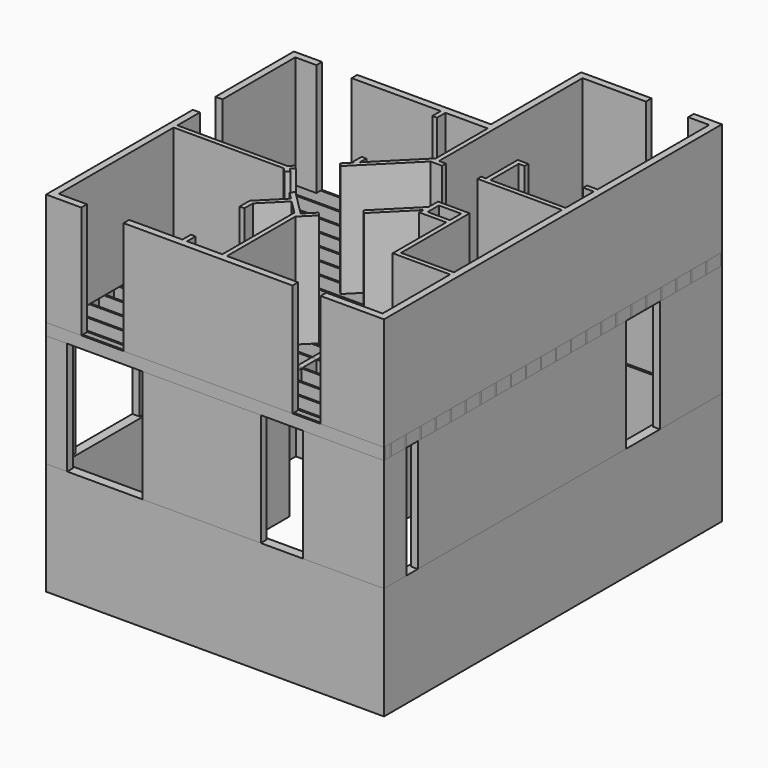
from build123d import *

# Parameters (mm, degrees)
F3_DEPTH  = 2438.4
F5_DEPTH  = 2438.4
F4_W      = 101.6
F4_H      = 1651.1016
F4_W_2    = 482.6
F4_H_2    = 304.8
F6_W      = 114.3
F6_H      = 254
F7_DEPTH  = 9144
F6_W_2    = 38.1
F8_W      = 38.1
F8_H      = 254
F9_DEPTH  = 7315.2
F11_DEPTH = 2438.4
F10_W     = 482.6
F10_H     = 304.8
F13_DEPTH = 5130.801


with BuildPart() as f3:
    # F2 (on Top) → F3 (new body)
    with BuildSketch(Plane.XY):
        Polygon((-4267.2, 0), (0, 0), (3048, 0), (3048, 9144), (0, 9144), (0, 6705.6), (-4267.2, 6705.6), align=None)
        Polygon((-4064, 6502.4), (203.2, 6502.4), (203.2, 8940.8), (2844.8, 8940.8), (2844.8, 203.2), (0, 203.2), (-4064, 203.2), align=None, mode=Mode.SUBTRACT)
    extrude(amount=-F3_DEPTH)


with BuildPart() as f5:
    # F4 (on face) → F5 (new body)
    with BuildSketch(Plane.XY):
        Polygon((-4267.2, 152.4), (-4267.2, 0), (-3810, 0), (-3810, 152.4), (-4114.8, 152.4), (-4114.8, 609.6), (-4267.2, 609.6), align=None)
    extrude(amount=F5_DEPTH)


with BuildPart() as f5b:
    # F4 (on face) → F5, piece 2 (new body)
    with BuildSketch(Plane.XY):
        Polygon((-4267.2, 6705.6), (-4267.2, 2336.8), (-4114.8, 2336.8), (-4114.8, 5232.4), (-3149.6, 5232.4), (-3149.6, 5334), (-4114.8, 5334), (-4114.8, 6553.2), (-2286, 6553.2), (-2286, 5334), (-2387.6, 5334), (-2387.6, 5232.4), (-2184.4, 5232.4), (-2184.4, 5334), (-2184.4, 6553.2), (-1879.6, 6553.2), (-1879.6, 6705.6), (-4114.8, 6705.6), align=None)
    extrude(amount=F5_DEPTH)


with BuildPart() as f5c:
    # F4 (on face) → F5, piece 3 (new body)
    with BuildSketch(Plane.XY):
        Polygon((0, 6705.6), (-1066.8, 6705.6), (-1066.8, 6553.2), (0, 6553.2), (152.4, 6553.2), (152.4, 8991.6), (2895.6, 8991.6), (2895.6, 7467.6), (3048, 7467.6), (3048, 8991.6), (3048, 9144), (152.4, 9144), (0, 9144), align=None)
    extrude(amount=F5_DEPTH)


with BuildPart() as f5d:
    # F4 (on face) → F5, piece 4 (new body)
    with BuildSketch(Plane.XY):
        Polygon((3048, 914.4), (3048, 6553.2), (2895.6, 6553.2), (2895.6, 5181.6), (1752.6, 5181.6), (1752.6, 5080.1016), (2895.6, 5080.1016), (2895.6, 914.4), align=None)
    extrude(amount=F5_DEPTH)


with BuildPart() as f5e:
    # F4 (on face) → F5, piece 5 (new body)
    with BuildSketch(Plane.XY):
        Polygon((-2184.4, 152.4), (-2184.4, 0), (381, 0), (381, 152.4), (152.4, 152.4), (152.4, 1066.8), (50.8, 1066.8), (50.8, 152.4), align=None)
    extrude(amount=F5_DEPTH)


with BuildPart() as f5f:
    # F4 (on face) → F5, piece 6 (new body)
    with BuildSketch(Plane.XY):
        Polygon((2895.6, 152.4), (1295.4, 152.4), (1295.4, 0), (3048, 0), (3048, 152.4), (3048, 609.6), (2895.6, 609.6), align=None)
    extrude(amount=F5_DEPTH)


with BuildPart() as f5g:
    # F4 (on face) → F5, piece 7 (new body)
    with BuildSketch(Plane.XY):
        with Locations((101.6, 3111.5508)):
            Rectangle(F4_W, F4_H)
    extrude(amount=F5_DEPTH)


with BuildPart() as f5h:
    # F4 (on face) → F5, piece 8 (new body)
    with BuildSketch(Plane.XY):
        Polygon((1752.6, 3937.1016), (1066.8, 3937.1016), (1066.8, 3276.8032), (1168.4, 3276.8032), (1168.4, 3429.2032), (1651, 3429.2032), (1651, 1473.2), (1168.4, 1473.2), (1168.4, 1655.9784), (1066.8, 1655.9784), (1066.8, 1371.6), (1752.6, 1371.6), align=None)
        with Locations((1409.7, 3683.1016)):
            Rectangle(F4_W_2, F4_H_2, mode=Mode.SUBTRACT)
    extrude(amount=F5_DEPTH)


with BuildPart() as f7:
    # F6 (on Front) → F7 (new body)
    with BuildSketch(Plane.XZ):
        with Locations((95.25, 2565.4)):
            Rectangle(F6_W, F6_H)
    extrude(amount=-F7_DEPTH)


with BuildPart() as f7b:
    # F6 (on Front) → F7, piece 2 (new body)
    with BuildSketch(Plane.XZ):
        with Locations((3028.95, 2565.4)):
            Rectangle(F6_W_2, F6_H)
    extrude(amount=-F7_DEPTH)


with BuildPart() as f7c:
    # F6 (on Front) → F7, piece 3 (new body)
    with BuildSketch(Plane.XZ):
        with Locations((-4248.15, 2565.4)):
            Rectangle(F6_W_2, F6_H)
    extrude(amount=-F7_DEPTH)

    # F8 (on face) → F9, piece 7 (join)
    with BuildSketch(Plane(origin=(-4267.2, 0, 0), x_dir=(0, -1, 0), z_dir=(-1, 0, 0))):
        with Locations((-6686.55, 2565.4)):
            Rectangle(F8_W, F8_H)
        with Locations((-6280.15, 2565.4)):
            Rectangle(F8_W, F8_H)
        with Locations((-5873.75, 2565.4)):
            Rectangle(F8_W, F8_H)
        with Locations((-5467.35, 2565.4)):
            Rectangle(F8_W, F8_H)
        with Locations((-5060.95, 2565.4)):
            Rectangle(F8_W, F8_H)
        with Locations((-4654.55, 2565.4)):
            Rectangle(F8_W, F8_H)
        with Locations((-4248.15, 2565.4)):
            Rectangle(F8_W, F8_H)
        with Locations((-3841.75, 2565.4)):
            Rectangle(F8_W, F8_H)
        with Locations((-3435.35, 2565.4)):
            Rectangle(F8_W, F8_H)
        with Locations((-3028.95, 2565.4)):
            Rectangle(F8_W, F8_H)
        with Locations((-2622.55, 2565.4)):
            Rectangle(F8_W, F8_H)
        with Locations((-2216.15, 2565.4)):
            Rectangle(F8_W, F8_H)
        with Locations((-1809.75, 2565.4)):
            Rectangle(F8_W, F8_H)
        with Locations((-1403.35, 2565.4)):
            Rectangle(F8_W, F8_H)
        with Locations((-996.95, 2565.4)):
            Rectangle(F8_W, F8_H)
        with Locations((-590.55, 2565.4)):
            Rectangle(F8_W, F8_H)
        with Locations((-184.15, 2565.4)):
            Rectangle(F8_W, F8_H)
        with Locations((-19.05, 2565.4)):
            Rectangle(F8_W, F8_H)
    extrude(amount=-F9_DEPTH)


with BuildPart() as f9:
    # F8 (on face) → F9 (new body)
    with BuildSketch(Plane(origin=(-4267.2, 0, 0), x_dir=(0, -1, 0), z_dir=(-1, 0, 0))):
        with Locations((-9124.95, 2565.4)):
            Rectangle(F8_W, F8_H)
    extrude(amount=-F9_DEPTH)


with BuildPart() as f9b:
    # F8 (on face) → F9, piece 2 (new body)
    with BuildSketch(Plane(origin=(-4267.2, 0, 0), x_dir=(0, -1, 0), z_dir=(-1, 0, 0))):
        with Locations((-8718.55, 2565.4)):
            Rectangle(F8_W, F8_H)
    extrude(amount=-F9_DEPTH)


with BuildPart() as f9c:
    # F8 (on face) → F9, piece 3 (new body)
    with BuildSketch(Plane(origin=(-4267.2, 0, 0), x_dir=(0, -1, 0), z_dir=(-1, 0, 0))):
        with Locations((-8312.15, 2565.4)):
            Rectangle(F8_W, F8_H)
    extrude(amount=-F9_DEPTH)


with BuildPart() as f9d:
    # F8 (on face) → F9, piece 4 (new body)
    with BuildSketch(Plane(origin=(-4267.2, 0, 0), x_dir=(0, -1, 0), z_dir=(-1, 0, 0))):
        with Locations((-7905.75, 2565.4)):
            Rectangle(F8_W, F8_H)
    extrude(amount=-F9_DEPTH)


with BuildPart() as f9e:
    # F8 (on face) → F9, piece 5 (new body)
    with BuildSketch(Plane(origin=(-4267.2, 0, 0), x_dir=(0, -1, 0), z_dir=(-1, 0, 0))):
        with Locations((-7499.35, 2565.4)):
            Rectangle(F8_W, F8_H)
    extrude(amount=-F9_DEPTH)


with BuildPart() as f9f:
    # F8 (on face) → F9, piece 6 (new body)
    with BuildSketch(Plane(origin=(-4267.2, 0, 0), x_dir=(0, -1, 0), z_dir=(-1, 0, 0))):
        with Locations((-7092.95, 2565.4)):
            Rectangle(F8_W, F8_H)
    extrude(amount=-F9_DEPTH)


with BuildPart() as f11:
    # F10 (on offset) → F11 (new body)
    with BuildSketch(Plane.XY.offset(2692.4)):
        Polygon((-4114.8, 4582.0584), (-4114.8, 6553.2), (-3657.6, 6553.2), (-3657.6, 6705.6), (-4267.2, 6705.6), (-4267.2, 4582.0584), align=None)
    extrude(amount=F11_DEPTH)


with BuildPart() as f11b:
    # F10 (on offset) → F11, piece 2 (new body)
    with BuildSketch(Plane.XY.offset(2692.4)):
        Polygon((-472.567, 2143.7854), (-1030.3052258163, 2701.5236258163), (-1102.0754327358, 2629.7534188967), (-940.4308225566, 2468.1088087174), (-1437.5638, 1970.975831274), (-1437.5638, 1700.3338174349), (-1336.0654, 1700.3338174349), (-1336.0654, 1928.9338174349), (-868.660615637, 2396.3386017979), (-574.0654, 2101.7433861608), (-574.0654, 152.4), (-472.567, 152.4), (-472.567, 2000.2449861608), (-185.2706461748, 2287.5413399861), (-257.0408530943, 2359.3115469057), align=None)
        Polygon((1066.8, 152.4), (-472.567, 152.4), (-574.0654, 152.4), (-1336.0654, 152.4), (-1336.0654, 381), (-1437.5638, 381), (-1437.5638, 152.4), (-2590.8, 152.4), (-2590.8, 0), (1066.8, 0), align=None)
    extrude(amount=F11_DEPTH)


with BuildPart() as f11c:
    # F10 (on offset) → F11, piece 3 (new body)
    with BuildSketch(Plane.XY.offset(2692.4)):
        Polygon((-4114.8, 3362.8584), (-4114.8, 3972.4584), (-4267.2, 3972.4584), (-4267.2, 0), (-3505.2, 0), (-3505.2, 152.4), (-4114.8, 152.4), (-4114.8, 3261.36), (-1733.6820138392, 3261.36), (-1640.8908, 3168.5687861608), (-1569.1205930804, 3240.3389930804), (-1640.8908, 3312.1092), (-1569.1205930804, 3383.8794069196), (-1640.8908, 3455.6496138392), (-1733.6820138392, 3362.8584), align=None)
    extrude(amount=F11_DEPTH)


with BuildPart() as f11d:
    # F10 (on offset) → F11, piece 4 (new body)
    with BuildSketch(Plane.XY.offset(2692.4)):
        Polygon((2895.6, 152.4), (1676.4, 152.4), (1676.4, 0), (3048, 0), (3048, 2081.784), (3048, 5003.9016), (3048, 6420.5906391144), (3048, 9144), (2438.4, 9144), (2438.4, 8991.6), (2895.6, 8991.6), (2895.6, 6420.5906391144), (2895.6, 5968.8984), (2667, 5968.8984), (2667, 5867.4), (2895.6, 5867.4), (2895.6, 5105.4), (1269.7968, 5105.4), (1269.7968, 5867.4), (1396.8984, 5867.4), (1396.8984, 5968.8984), (1168.2984, 5968.8984), (1168.2984, 5105.4), (1066.8, 5105.4), (1066.8, 5003.9016), (2895.6, 5003.9016), (2895.6, 2081.784), (1752.6, 2081.784), (1752.6, 3937.1016), (1066.8, 3937.1016), (1066.8, 3683.1524), (281.7745141698, 2898.1269141698), (353.5447210894, 2826.3567072502), (1066.8, 3539.6119861608), (1066.8, 3429.2032), (1652.016, 3429.2032), (1652.016, 1981.2), (2895.6, 1981.2), align=None)
        with Locations((1409.7, 3683.1016)):
            Rectangle(F10_W, F10_H, mode=Mode.SUBTRACT)
    extrude(amount=F11_DEPTH)


with BuildPart() as f11e:
    # F10 (on offset) → F11, piece 5 (new body)
    with BuildSketch(Plane.XY.offset(2692.4)):
        Polygon((0, 6705.6), (-2895.6, 6705.6), (-2895.6, 6553.2), (-964.9968, 6553.2), (-964.9968, 6324.6), (-863.4984, 6324.6), (-863.4984, 6553.2), (50.9016, 6553.2), (50.9016, 5147.4420138392), (-863.4984, 4233.0420138392), (-863.4984, 4222.7175825651), (-868.660615637, 4227.8797982021), (-940.4308225566, 4156.1095912826), (-1102.0754327359, 3994.4649811033), (-1030.3052258163, 3922.6947741837), (50.9016, 5003.9016), (304.8, 5003.9016), (304.8, 5105.4), (152.4, 5105.4), (152.4, 6705.6), (152.4, 8991.6), (1524, 8991.6), (1524, 9144), (0, 9144), align=None)
        Polygon((-863.4984, 4222.7175825651), (-863.4984, 4233.0420138392), (-868.660615637, 4227.8797982021), align=None)
        Polygon((-868.660615637, 4227.8797982021), (-863.4984, 4233.0420138392), (-863.4984, 4409.275568726), (-964.9968, 4409.275568726), (-964.9968, 4180.675568726), (-940.4308225566, 4156.1095912826), align=None)
    extrude(amount=F11_DEPTH)


with BuildPart() as f13_tool:
    # F12 (on Top) → F13 (new body, through all)
    with BuildSketch(Plane.XY):
        Polygon((-8839.2000267029, 11277.6000267029), (-8839.2000267029, -4572.0000267029), (7620.0000267029, -4572.0000267029), (7620.0000267029, 13716.0000267029), (-4572.0000267029, 13716.0000267029), (-4572.0000267029, 11277.6000267029), align=None)
        Polygon((3048, 0), (-4267.2, 0), (-4267.2, 6705.6), (0, 6705.6), (0, 9144), (3048, 9144), align=None, mode=Mode.SUBTRACT)
    extrude(amount=F13_DEPTH)


with BuildPart() as f7c_1:
    add(f7c.part)

    # F13: cut by f13_tool
    add(f13_tool.part, mode=Mode.SUBTRACT)


with BuildPart() as f9_1:
    add(f9.part)

    # F13: cut by f13_tool
    add(f13_tool.part, mode=Mode.SUBTRACT)


with BuildPart() as f9b_1:
    add(f9b.part)

    # F13: cut by f13_tool
    add(f13_tool.part, mode=Mode.SUBTRACT)


with BuildPart() as f9c_1:
    add(f9c.part)

    # F13: cut by f13_tool
    add(f13_tool.part, mode=Mode.SUBTRACT)


with BuildPart() as f9d_1:
    add(f9d.part)

    # F13: cut by f13_tool
    add(f13_tool.part, mode=Mode.SUBTRACT)


with BuildPart() as f9e_1:
    add(f9e.part)

    # F13: cut by f13_tool
    add(f13_tool.part, mode=Mode.SUBTRACT)


with BuildPart() as f9f_1:
    add(f9f.part)

    # F13: cut by f13_tool
    add(f13_tool.part, mode=Mode.SUBTRACT)


solid = Compound([f3.part, f5.part, f5b.part, f5c.part, f5d.part, f5e.part, f5f.part, f5g.part, f5h.part, f7.part, f7b.part, f11.part, f11b.part, f11c.part, f11d.part, f11e.part, f7c_1.part, f9_1.part, f9b_1.part, f9c_1.part, f9d_1.part, f9e_1.part, f9f_1.part])
